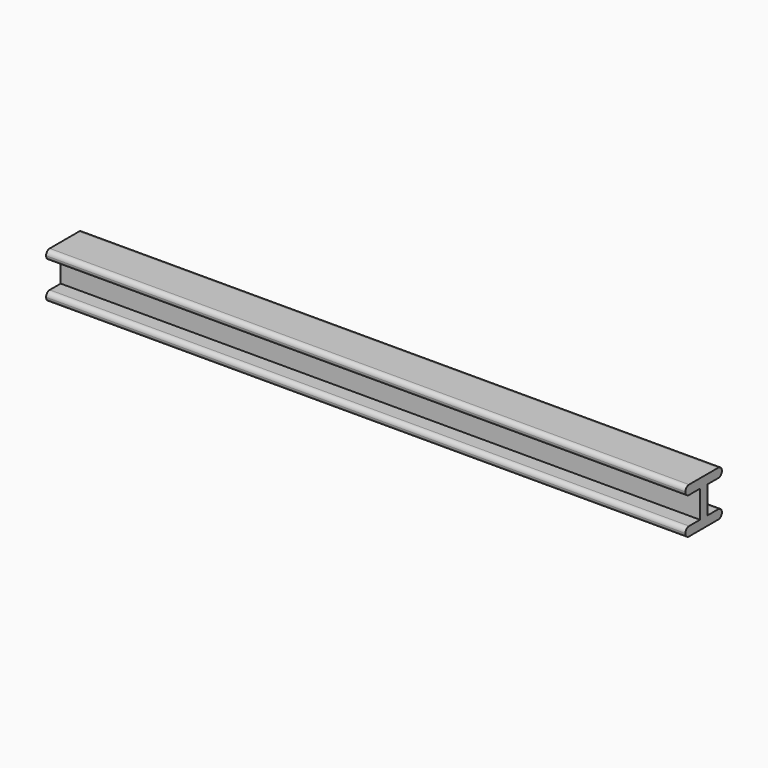
from build123d import *

# Parameters (mm, degrees)
F0_W     = 177.8
F0_H     = 12.7
F1_DEPTH = 12.7
F2_R     = 1.27
F3_W     = 5.08
F3_H     = 7.62
F4_DEPTH = 177.8
F5_R     = 1.26999


# Not quite as in the source:
# - a fillet or chamfer is up to 0.001 mm smaller than in the source, because OpenCascade refuses the exact size


with BuildPart() as f1:
    # F0 (on Top) → F1 (new body)
    with BuildSketch(Plane.XY):
        Rectangle(F0_W, F0_H)
    extrude(amount=F1_DEPTH)

    # F2
    f2_edges = [f1.edges().sort_by_distance(p)[0] for p in [
        (0, 6.35, 0),
        (0, 6.35, 12.7),
        (0, -6.35, 12.7),
        (0, -6.35, 0),
    ]]
    fillet(f2_edges, radius=F2_R)

    # F3 (on face) → F4 (cut)
    with BuildSketch(Plane.YZ.offset(88.9)):
        with Locations((-3.81, 6.35)):
            Rectangle(F3_W, F3_H)
        with Locations((3.81, 6.35)):
            Rectangle(F3_W, F3_H)
    extrude(amount=-F4_DEPTH, mode=Mode.SUBTRACT)

    # F5 (radius 1.27 in the source; OpenCascade refuses exactly that, so slightly less here)
    f5_edges = [f1.edges().sort_by_distance(p)[0] for p in [
        (0, 6.35, 10.16),
        (0, 6.35, 2.54),
        (0, -6.35, 10.16),
        (0, -6.35, 2.54),
    ]]
    fillet(f5_edges, radius=F5_R)


solid = f1.part
